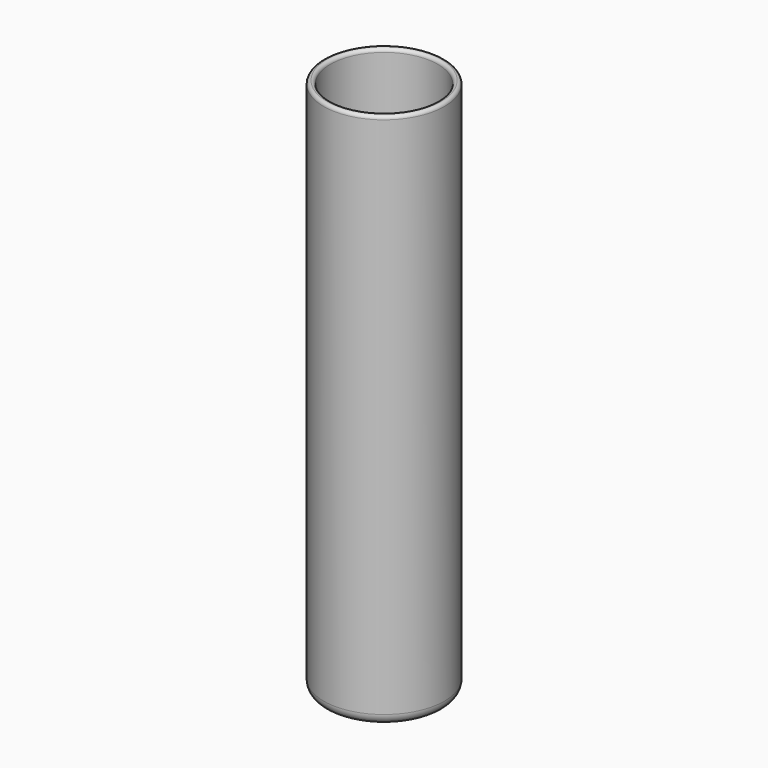
from build123d import *

# Parameters (mm, degrees)
F0_W = 14.2875
F0_H = 127
F2_T = -1.5875
F3_R = 2.54
F4_R = 0.79374


# Not quite as in the source:
# - a fillet or chamfer is up to 0.001 mm smaller than in the source, because OpenCascade refuses the exact size


with BuildPart() as f1:
    # F0 (on Front) → F1 (revolve)
    with BuildSketch(Plane.XZ):
        with Locations((7.14375, 0)):
            Rectangle(F0_W, F0_H)
    revolve(axis=Axis((0, 0, 0), (0, 0, -1)))

    # F2
    f2_openings = [f1.faces().sort_by_distance(p)[0] for p in [
        (0, 0, 63.5),
    ]]
    offset(amount=F2_T, openings=f2_openings)

    # F3
    f3_edges = [f1.edges().sort_by_distance(p)[0] for p in [
        (-14.2875, 0, -63.5),
    ]]
    fillet(f3_edges, radius=F3_R)

    # F4 (radius 0.79375 in the source; OpenCascade refuses exactly that, so slightly less here)
    f4_edges = [f1.edges().sort_by_distance(p)[0] for p in [
        (-14.2875, 0, 63.5),
        (-12.7, 0, 63.5),
    ]]
    fillet(f4_edges, radius=F4_R)


solid = f1.part
